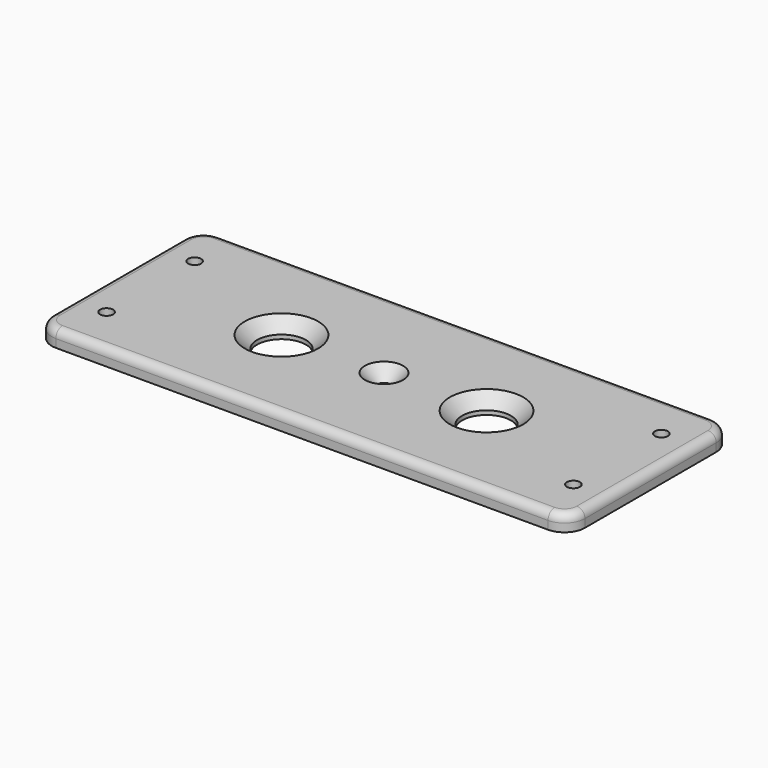
from build123d import *

# Parameters (mm, degrees)
F1_DEPTH = 4
F2_R     = 5.9436
F2_R_2   = 1.6637
F2_R_3   = 1.5875
F3_DEPTH = 25
F4_R     = 5
F5_R     = 2
F6_SIZE  = 3
F7_SIZE  = 3


# Not quite as in the source:
# - a feature names something its author has since deleted; it is built from what else it names


with BuildPart() as f1:
    # F0 (on Top) → F1 (new body)
    with BuildSketch(Plane.XY):
        Polygon((65, -25), (65, 25), (33, 25), (-33, 25), (-65, 25), (-65, -25), align=None)
    extrude(amount=F1_DEPTH)

    # F2 (on Top) → F3 (cut)
    with BuildSketch(Plane.XY):
        with Locations((-25, 0)):
            Circle(F2_R)
        Circle(F2_R_2)
        with Locations((25, 0)):
            Circle(F2_R)
        with Locations((-56.9125, 13.4125)):
            Circle(F2_R_3)
        with Locations((-56.9125, -13.4125)):
            Circle(F2_R_3)
        with Locations((56.9125, 13.4125)):
            Circle(F2_R_3)
        with Locations((56.9125, -13.4125)):
            Circle(F2_R_3)
    extrude(amount=F3_DEPTH, mode=Mode.SUBTRACT)

    # F4
    f4_edges = [f1.edges().sort_by_distance(p)[0] for p in [
        (-65, -25, 2),
        (65, -25, 2),
        (65, 25, 2),
        (-65, 25, 2),
    ]]
    fillet(f4_edges, radius=F4_R)

    # F5
    f5_edges = [f1.edges().sort_by_distance(p)[0] for p in [
        (-65, 0, 4),
    ]]
    fillet(f5_edges, radius=F5_R)

    # F6
    f6_edges = [f1.edges().sort_by_distance(p)[0] for p in [
        (-30.9436, 0, 4),
        (19.0564, 0, 4),
    ]]
    chamfer(f6_edges, length=F6_SIZE)

    # F7
    f7_edges = [f1.edges().sort_by_distance(p)[0] for p in [
        (-1.6637, 0, 4),
    ]]
    chamfer(f7_edges, length=F7_SIZE)


solid = f1.part
